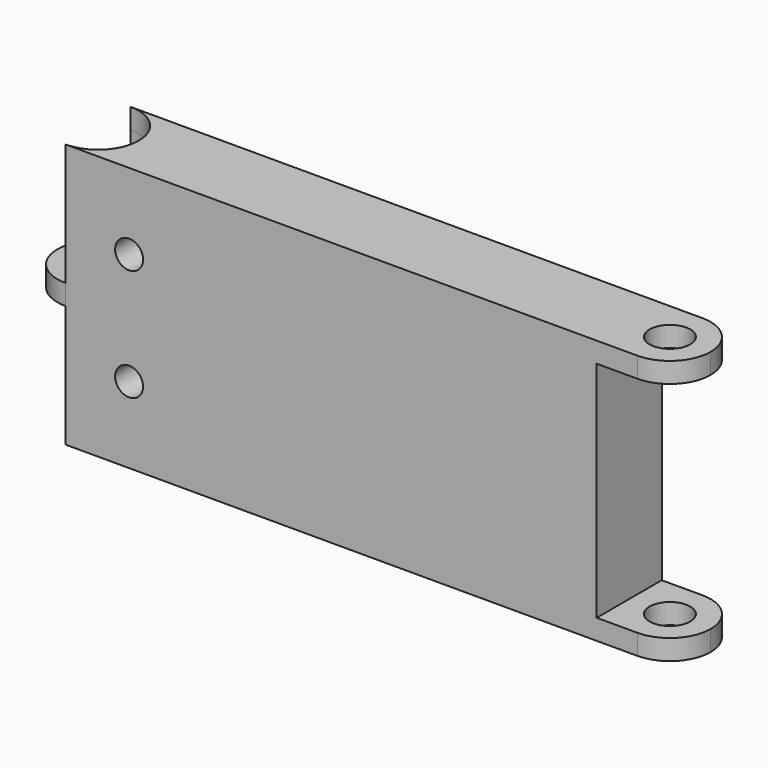
from build123d import *

# Parameters (mm, degrees)
F0_R      = 1.6
F1_DEPTH  = 1.6
F4_DEPTH  = 8
F5_R      = 1.6
F6_DEPTH  = 1.6
F8_DEPTH  = 8
F9_R      = 1.6
F10_DEPTH = 1.6
F12_D     = 2.2
F12_DEPTH = 2.4
F12_TIP   = 0.6609466809


with BuildPart() as f1:
    # F0 (on Top) → F1 (new body)
    with BuildSketch(Plane.XY):
        with BuildLine():
            Line((19.3, 3.2), (-22.5, 3.2))
            ThreePointArc((-22.5, 3.2), (-20.2372583002, 2.2627416998), (-19.3, 0))
            ThreePointArc((-19.3, 0), (-20.2372583002, -2.2627416998), (-22.5, -3.2))
            Line((-22.5, -3.2), (19.3, -3.2))
            Line((19.3, -3.2), (19.3, 0))
            Line((19.3, 0), (19.3, 3.2))
        make_face()
        with BuildLine():
            Line((22.5, 3.2), (19.3, 3.2))
            Line((19.3, 3.2), (19.3, 0))
            ThreePointArc((19.3, 0), (20.2372583002, 2.2627416998), (22.5, 3.2))
        make_face()
        with BuildLine():
            ThreePointArc((25.7, 0), (24.7627416998, 2.2627416998), (22.5, 3.2))
            ThreePointArc((22.5, 3.2), (20.2372583002, 2.2627416998), (19.3, 0))
            ThreePointArc((19.3, 0), (20.2372583002, -2.2627416998), (22.5, -3.2))
            ThreePointArc((22.5, -3.2), (24.7627416998, -2.2627416998), (25.7, 0))
        make_face()
        with Locations((22.5, 0)):
            Circle(F0_R, mode=Mode.SUBTRACT)
        with BuildLine():
            Line((19.3, 0), (19.3, -3.2))
            Line((19.3, -3.2), (22.5, -3.2))
            ThreePointArc((22.5, -3.2), (20.2372583002, -2.2627416998), (19.3, 0))
        make_face()
    extrude(amount=F1_DEPTH)

    # F3 (on offset) → F4 (join)
    with BuildSketch(Plane.XY.offset(1.6)):
        with BuildLine():
            ThreePointArc((-22.5, 3.2), (-20.2372583002, 2.2627416998), (-19.3, 0))
            ThreePointArc((-19.3, 0), (-20.2372583002, -2.2627416998), (-22.5, -3.2))
            Line((-22.5, -3.2), (19.3, -3.2))
            Line((19.3, -3.2), (19.3, 0))
            Line((19.3, 0), (19.3, 3.2))
            Line((19.3, 3.2), (-22.5, 3.2))
        make_face()
    extrude(amount=F4_DEPTH)

    # F5 (on face) → F6 (join)
    with BuildSketch(Plane.XY.offset(9.6)):
        with BuildLine():
            Line((-22.5, -3.2), (19.3, -3.2))
            Line((19.3, -3.2), (19.3, 3.2))
            Line((19.3, 3.2), (-22.5, 3.2))
            ThreePointArc((-22.5, 3.2), (-20.2372583002, 2.2627416998), (-19.3, 0))
            ThreePointArc((-19.3, 0), (-20.2372583002, -2.2627416998), (-22.5, -3.2))
        make_face()
        with BuildLine():
            ThreePointArc((-22.5, 3.2), (-25.7, 0), (-22.5, -3.2))
            ThreePointArc((-22.5, -3.2), (-20.2372583002, -2.2627416998), (-19.3, 0))
            ThreePointArc((-19.3, 0), (-20.2372583002, 2.2627416998), (-22.5, 3.2))
        make_face()
        with Locations((-22.5, 0)):
            Circle(F5_R, mode=Mode.SUBTRACT)
    extrude(amount=F6_DEPTH)

    # F7 (on face) → F8 (join)
    with BuildSketch(Plane.XY.offset(11.2)):
        with BuildLine():
            Line((-22.5, -3.2), (19.3, -3.2))
            Line((19.3, -3.2), (19.3, 0))
            Line((19.3, 0), (19.3, 3.2))
            Line((19.3, 3.2), (-22.5, 3.2))
            ThreePointArc((-22.5, 3.2), (-20.2372583002, 2.2627416998), (-19.3, 0))
            ThreePointArc((-19.3, 0), (-20.2372583002, -2.2627416998), (-22.5, -3.2))
        make_face()
    extrude(amount=F8_DEPTH)

    # F9 (on face) → F10 (join)
    with BuildSketch(Plane.XY.offset(19.2)):
        with BuildLine():
            Line((19.3, -3.2), (19.3, 0))
            Line((19.3, 0), (19.3, 3.2))
            Line((19.3, 3.2), (-22.5, 3.2))
            ThreePointArc((-22.5, 3.2), (-19.3, 0), (-22.5, -3.2))
            Line((-22.5, -3.2), (19.3, -3.2))
        make_face()
        with BuildLine():
            ThreePointArc((19.3, 0), (20.2372583002, 2.2627416998), (22.5, 3.2))
            Line((22.5, 3.2), (19.3, 3.2))
            Line((19.3, 3.2), (19.3, 0))
        make_face()
        with BuildLine():
            ThreePointArc((22.5, -3.2), (24.7627416998, -2.2627416998), (25.7, 0))
            ThreePointArc((25.7, 0), (24.7627416998, 2.2627416998), (22.5, 3.2))
            ThreePointArc((22.5, 3.2), (20.2372583002, 2.2627416998), (19.3, 0))
            ThreePointArc((19.3, 0), (20.2372583002, -2.2627416998), (22.5, -3.2))
        make_face()
        with Locations((22.5, 0)):
            Circle(F9_R, mode=Mode.SUBTRACT)
        with BuildLine():
            Line((19.3, -3.2), (22.5, -3.2))
            ThreePointArc((22.5, -3.2), (20.2372583002, -2.2627416998), (19.3, 0))
            Line((19.3, 0), (19.3, -3.2))
        make_face()
    extrude(amount=F10_DEPTH)

    # F12
    with Locations(Plane.XZ.offset(3.2)):
        with Locations((-17.5, 14.8), (-17.5, 6)):
            Hole(F12_D / 2, depth=F12_DEPTH)
            with Locations((0, 0, -(F12_DEPTH + F12_TIP / 2))):  # 118° drill point
                Cone(0, F12_D / 2, F12_TIP, mode=Mode.SUBTRACT)


solid = f1.part
